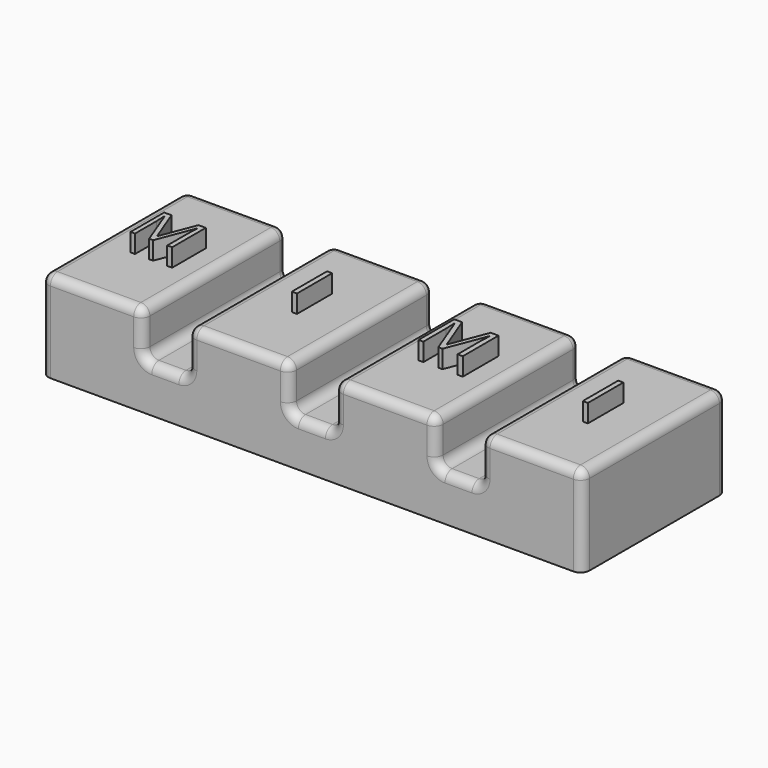
from build123d import *

# Parameters (mm, degrees)
F0_W           = 76.2
F0_H           = 25.4
F1_DEPTH       = 12.7
F2_W           = 6.35
F2_H           = 12.7
F3_DEPTH       = 25.401
F4_R           = 1.27
F5_T           = -2.54
F6_TEXT_SIZE   = 8.8130178887
F6_TEXT_SIZE_2 = 8.294605262
F6_TEXT_SIZE_3 = 8.6787803512
F6_TEXT_SIZE_4 = 8.734524858
F7_DEPTH       = 2.54


# Not quite as in the source:
# - Text() gives the source's letters only with a copy of the font that has no kerning and outlines rounded to 1/6400 em; it was checked with that copy


with BuildPart() as f1:
    # F0 (on Top) → F1 (new body)
    with BuildSketch(Plane.XY):
        Rectangle(F0_W, F0_H)
    extrude(amount=F1_DEPTH)

    # F2 (on face) → F3 (cut, through all)
    with BuildSketch(Plane(origin=(0, 12.7, 0), x_dir=(-1, 0, 0), z_dir=(0, 1, 0))):
        with Locations((0, 12.7)):
            Rectangle(F2_W, F2_H)
        with Locations((-20.6502, 12.7)):
            Rectangle(F2_W, F2_H)
        with Locations((20.6502, 12.7)):
            Rectangle(F2_W, F2_H)
    extrude(amount=-F3_DEPTH, mode=Mode.SUBTRACT)

    # F4
    f4_edges = [f1.edges().sort_by_distance(p)[0] for p in [
        (10.3251, -12.7, 12.7),
        (3.175, 0, 12.7),
        (10.3251, 12.7, 12.7),
        (17.4752, 0, 12.7),
        (30.9626, -12.7, 12.7),
        (23.8252, 0, 12.7),
        (30.9626, 12.7, 12.7),
        (38.1, 0, 12.7),
        (-10.3251, -12.7, 12.7),
        (-17.4752, 0, 12.7),
        (-10.3251, 12.7, 12.7),
        (-3.175, 0, 12.7),
        (-30.9626, -12.7, 12.7),
        (-38.1, 0, 12.7),
        (-30.9626, 12.7, 12.7),
        (-23.8252, 0, 12.7),
        (20.6502, 12.7, 6.35),
        (17.4752, 0, 6.35),
        (20.6502, -12.7, 6.35),
        (23.8252, 0, 6.35),
        (0, 12.7, 6.35),
        (-3.175, 0, 6.35),
        (0, -12.7, 6.35),
        (3.175, 0, 6.35),
        (-20.6502, 12.7, 6.35),
        (-23.8252, 0, 6.35),
        (-20.6502, -12.7, 6.35),
        (-17.4752, 0, 6.35),
        (-38.1, 12.7, 6.35),
        (38.1, 12.7, 6.35),
        (38.1, -12.7, 6.35),
        (-38.1, -12.7, 6.35),
        (23.8252, -12.7, 9.525),
        (17.4752, -12.7, 9.525),
        (3.175, -12.7, 9.525),
        (-3.175, -12.7, 9.525),
        (-17.4752, -12.7, 9.525),
        (-23.8252, -12.7, 9.525),
        (-23.8252, 12.7, 9.525),
        (-17.4752, 12.7, 9.525),
        (-3.175, 12.7, 9.525),
        (3.175, 12.7, 9.525),
        (17.4752, 12.7, 9.525),
        (23.8252, 12.7, 9.525),
    ]]
    fillet(f4_edges, radius=F4_R)

    # F5
    f5_openings = [f1.faces().sort_by_distance(p)[0] for p in [
        (0, 0, 0),
    ]]
    offset(amount=F5_T, openings=f5_openings)

    # F6 (on face) → F7 (join)
    with BuildSketch(Plane.XY.offset(12.7)):
        with Locations((6.5058828332, -3.1325841264)):
            Text('M', F6_TEXT_SIZE, font='Open Sans', text_align=(TextAlign.LEFT, TextAlign.BOTTOM))
        with Locations((-34.2538058758, -2.8339782148)):
            Text('M', F6_TEXT_SIZE_2, font='Open Sans', text_align=(TextAlign.LEFT, TextAlign.BOTTOM))
        with Locations((-11.5443523973, -2.8553474986)):
            Text('I', F6_TEXT_SIZE_3, font='Open Sans', text_align=(TextAlign.LEFT, TextAlign.BOTTOM))
        with Locations((29.7185461968, -3.2251655357)):
            Text('I', F6_TEXT_SIZE_4, font='Open Sans', text_align=(TextAlign.LEFT, TextAlign.BOTTOM))
    extrude(amount=F7_DEPTH)


solid = f1.part
